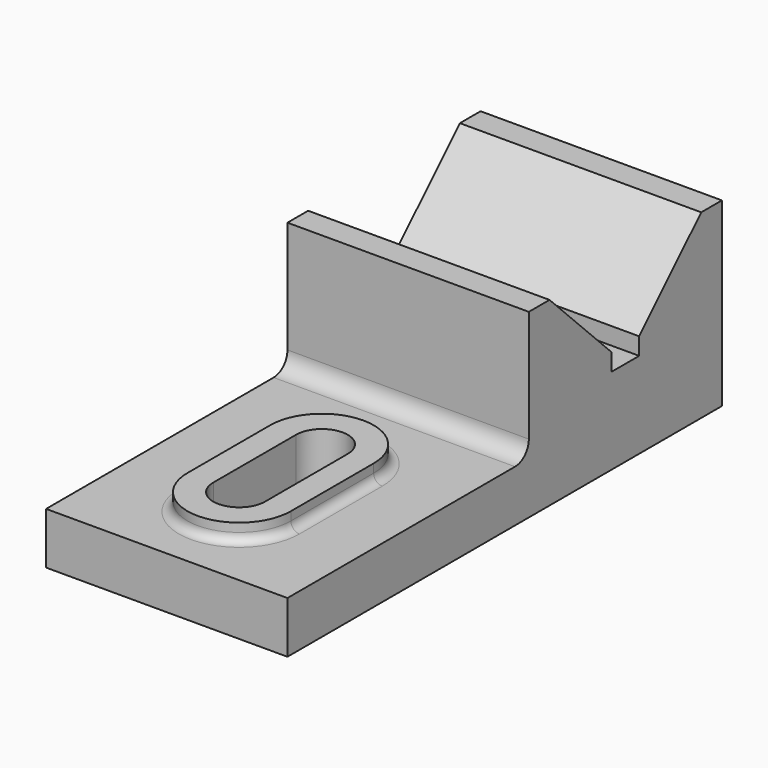
from build123d import *

# Parameters (mm, degrees)
F1_DEPTH = 88.9
F3_DEPTH = 6.35
F4_DEPTH = 19.05
F5_R     = 3.175


# Not quite as in the source:
# - a length typed as a fraction of an inch, garbled in the dataset ("3 / 203.2 mm" for 3/8 in), is restored


with BuildPart() as f1:
    # F0 (on Right) → F1 (new body)
    with BuildSketch(Plane.YZ):
        with BuildLine():
            Line((-61.4579357207, 19.05), (-61.4579357207, 66.675))
            Line((-61.4579357207, 66.675), (-70.9829357207, 66.675))
            Line((-70.9829357207, 66.675), (-99.5579357207, 38.1))
            Line((-99.5579357207, 38.1), (-99.5579357207, 31.75))
            Line((-99.5579357207, 31.75), (-112.2579357207, 31.75))
            Line((-112.2579357207, 31.75), (-112.2579357207, 38.1))
            Line((-112.2579357207, 38.1), (-140.8329357207, 66.675))
            Line((-140.8329357207, 66.675), (-150.3579357207, 66.675))
            Line((-150.3579357207, 66.675), (-150.3579357207, 25.4))
            ThreePointArc((-150.3579357207, 25.4), (-152.2178076601, 20.9098719395), (-156.7079357207, 19.05))
            Line((-156.7079357207, 19.05), (-261.4829357207, 19.05))
            Line((-261.4829357207, 19.05), (-261.4829357207, 0))
            Line((-261.4829357207, 0), (-150.3579357207, 0))
            Line((-150.3579357207, 0), (-140.8329357207, 0))
            Line((-140.8329357207, 0), (-74.1579357207, 0))
            Line((-74.1579357207, 0), (-70.9829357207, 0))
            Line((-70.9829357207, 0), (-61.4579357207, 0))
            Line((-61.4579357207, 0), (-61.4579357207, 19.05))
        make_face()
    extrude(amount=-F1_DEPTH)

    # F2 (on face) → F3 (join)
    with BuildSketch(Plane.XY.offset(19.05)):
        with BuildLine():
            Line((-25.4, -228.1454357207), (-25.4, -190.0454357207))
            ThreePointArc((-25.4, -190.0454357207), (-44.45, -170.9954357207), (-63.5, -190.0454357207))
            Line((-63.5, -190.0454357207), (-63.5, -228.1454357207))
            ThreePointArc((-63.5, -228.1454357207), (-44.45, -247.1954357207), (-25.4, -228.1454357207))
        make_face()
        with BuildLine():
            ThreePointArc((-34.925, -228.1454357207), (-44.45, -237.6704357207), (-53.975, -228.1454357207))
            Line((-53.975, -228.1454357207), (-53.975, -190.0454357207))
            ThreePointArc((-53.975, -190.0454357207), (-44.45, -180.5204357207), (-34.925, -190.0454357207))
            Line((-34.925, -190.0454357207), (-34.925, -228.1454357207))
        make_face(mode=Mode.SUBTRACT)
    extrude(amount=F3_DEPTH)

    # F4 (cut): a face of the model
    f4_faces = [f1.faces().sort_by_distance(p)[0] for p in [
        (-44.45, -209.0954357207, 19.05),
    ]]
    extrude(f4_faces, amount=-F4_DEPTH, mode=Mode.SUBTRACT)

    # F5
    f5_edges = [f1.edges().sort_by_distance(p)[0] for p in [
        (-63.5, -209.095436, 19.05),
    ]]
    fillet(f5_edges, radius=F5_R)


solid = f1.part
